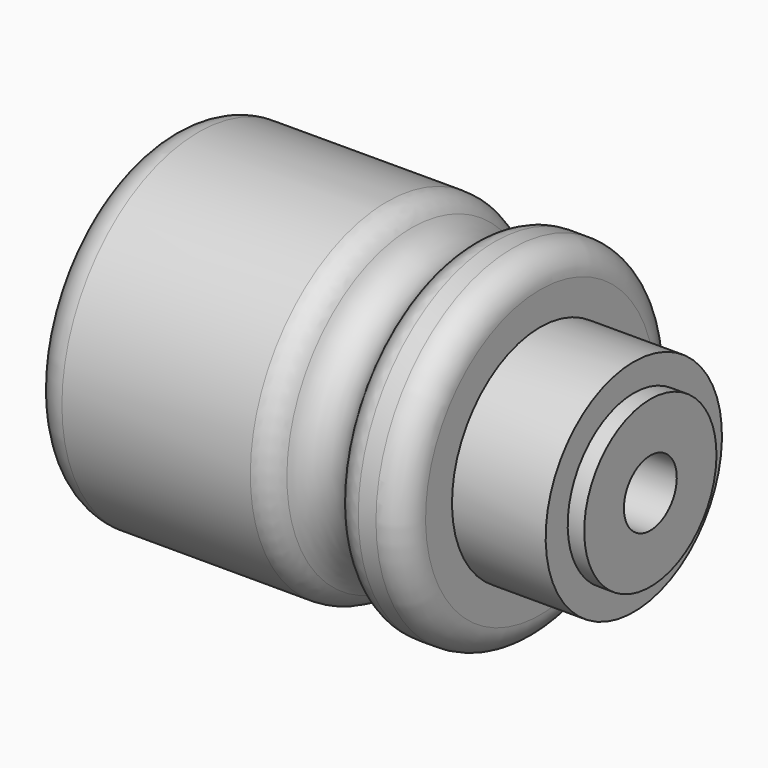
from build123d import *

# Parameters (mm, degrees)
F4_R = 5.99999
F5_R = 5
F6_R = 5


# Not quite as in the source:
# - a fillet or chamfer is up to 0.001 mm smaller than in the source, because OpenCascade refuses the exact size


with BuildPart() as f1:
    # F0 (on Front) → F1 (revolve)
    with BuildSketch(Plane.XZ):
        with BuildLine():
            Line((0, 31), (0, 0))
            Line((0, 0), (88, 0))
            Line((88, 0), (88, 15))
            Line((88, 15), (85, 15))
            Line((85, 15), (85, 20))
            Line((85, 20), (68, 20))
            Line((68, 20), (68, 31))
            Line((68, 31), (56, 31))
            ThreePointArc((56, 31), (50, 25), (44, 31))
            Line((44, 31), (0, 31))
        make_face()
    revolve(axis=Axis((44, 0, 0), (-1, 0, 0)))

    # F2 (on Front) → F3 (revolve, cut)
    with BuildSketch(Plane.XZ):
        Polygon((0, 25), (0, 0), (88, 0), (88, 6), (30, 6), (30, 16), (22, 16), (22, 20.5), (16.5, 20.5), (16.5, 12.5), (13.5, 12.5), (13.5, 16), (1.5, 16), (1.5, 25), align=None)
    revolve(axis=Axis((44.884205035, 0, 0), (1, 0, 0)), mode=Mode.SUBTRACT)

    # F4 (radius 6 in the source; OpenCascade refuses exactly that, so slightly less here)
    f4_edges = [f1.edges().sort_by_distance(p)[0] for p in [
        (0, 0, -31),
    ]]
    fillet(f4_edges, radius=F4_R)

    # F5
    f5_edges = [f1.edges().sort_by_distance(p)[0] for p in [
        (44, 0, -31),
        (56, 0, -31),
    ]]
    fillet(f5_edges, radius=F5_R)

    # F6
    f6_edges = [f1.edges().sort_by_distance(p)[0] for p in [
        (68, 0, -31),
    ]]
    fillet(f6_edges, radius=F6_R)


solid = f1.part
